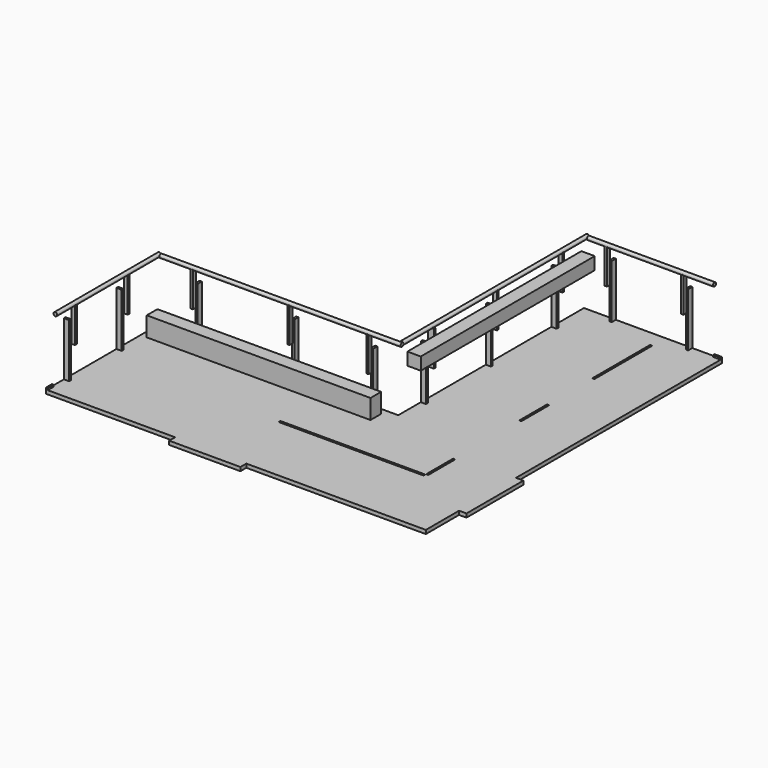
from build123d import *

# Parameters (mm, degrees)
F1_DEPTH  = 25.4
F2_W      = 30
F2_H      = 70
F2_W_2    = 70
F2_H_2    = 30
F3_DEPTH  = 750
F5_W      = 50
F5_H      = 30
F6_DEPTH  = 470
F5_W_2    = 30
F5_H_2    = 50
F7_R      = 25
F8_DEPTH  = 1700
F9_R      = 25
F10_DEPTH = 3130
F11_R     = 25
F12_DEPTH = 3250
F13_R     = 25
F14_DEPTH = 1750
F16_W     = 25
F16_H     = 970
F17_DEPTH = 3
F16_H_2   = 465
F16_W_2   = 1950
F16_H_3   = 25
F16_H_4   = 450
F18_DEPTH = 25
F19_W     = 100
F19_H     = 22
F19_W_2   = 22
F19_H_2   = 100
F20_DEPTH = 25
F21_DEPTH = 25
F22_W     = 2931.857542173
F22_H     = 168.5780864702
F23_DEPTH = 180
F24_W     = 3016.7315006256
F24_H     = 261.820666492
F25_DEPTH = 180


with BuildPart() as f1:
    # F0 (on Top) → F1 (new body)
    with BuildSketch(Plane.XY):
        Polygon((-2420, 0), (0, 0), (0, 560), (100, 560), (100, 1520), (0, 1520), (0, 4990), (-1860, 4990), (-1860, 1860), (-5120, 1860), (-5120, 0), (-3380, 0), (-3380, -100), (-2420, -100), align=None)
    extrude(amount=F1_DEPTH)

    # F2 (on face) → F3 (join)
    with BuildSketch(Plane.XY.offset(25.4)):
        with Locations((-415, 4955)):
            Rectangle(F2_W, F2_H)
        with Locations((-1825, 4455)):
            Rectangle(F2_W_2, F2_H_2)
        with Locations((-1825, 2255)):
            Rectangle(F2_W_2, F2_H_2)
        with Locations((-2156.2518024445, 1825)):
            Rectangle(F2_W, F2_H)
        with Locations((-3220.6851100922, 1825)):
            Rectangle(F2_W, F2_H)
        with Locations((-4523.8569831848, 1825)):
            Rectangle(F2_W, F2_H)
        with Locations((-1445, 4955)):
            Rectangle(F2_W, F2_H)
        with Locations((-5085, 315)):
            Rectangle(F2_W_2, F2_H_2)
        with Locations((-1825, 3350)):
            Rectangle(F2_W_2, F2_H_2)
        with Locations((-5085, 1201.3461732864)):
            Rectangle(F2_W_2, F2_H_2)
    extrude(amount=F3_DEPTH)

    # F2 (on face) → F18 (join)
    with BuildSketch(Plane.XY.offset(25.4)):
        Polygon((-430, 4920), (-430, 4990), (-1430, 4990), (-1430, 4920), (-1460, 4920), (-1460, 4990), (-1860, 4990), (-1860, 4470), (-1790, 4470), (-1790, 4440), (-1860, 4440), (-1860, 3365), (-1790, 3365), (-1790, 3335), (-1860, 3335), (-1860, 2270), (-1790, 2270), (-1790, 2240), (-1860, 2240), (-1860, 1860), (-2141.2518024445, 1860), (-2141.2518024445, 1790), (-2171.2518024445, 1790), (-2171.2518024445, 1860), (-3205.6851100922, 1860), (-3205.6851100922, 1790), (-3235.6851100922, 1790), (-3235.6851100922, 1860), (-4508.8569831848, 1860), (-4508.8569831848, 1790), (-4538.8569831848, 1790), (-4538.8569831848, 1860), (-5120, 1860), (-5120, 1216.3461732864), (-5050, 1216.3461732864), (-5050, 1186.3461732864), (-5120, 1186.3461732864), (-5120, 330), (-5050, 330), (-5050, 300), (-5120, 300), (-5120, 0), (-3380, 0), (-3380, -100), (-2420, -100), (-2420, 0), (0, 0), (0, 560), (100, 560), (100, 1520), (0, 1520), (0, 4990), (-400, 4990), (-400, 4920), align=None)
    extrude(amount=F18_DEPTH)

    # F19 (on face) → F20 (join)
    with BuildSketch(Plane.XY.offset(50.4)):
        with Locations((-50, 4979)):
            Rectangle(F19_W, F19_H)
        with Locations((-5109, 50)):
            Rectangle(F19_W_2, F19_H_2)
    extrude(amount=F20_DEPTH)


with BuildPart() as f6:
    # F5 (on offset) → F6 (new body)
    with BuildSketch(Plane.XY.offset(505.4)):
        with Locations((-1735, 4455)):
            Rectangle(F5_W, F5_H)
    extrude(amount=F6_DEPTH)



with BuildPart() as f6b:
    # F5 (on offset) → F6, piece 2 (new body)
    with BuildSketch(Plane.XY.offset(505.4)):
        with Locations((-1445, 4865)):
            Rectangle(F5_W_2, F5_H_2)
    extrude(amount=F6_DEPTH)



with BuildPart() as f6c:
    # F5 (on offset) → F6, piece 3 (new body)
    with BuildSketch(Plane.XY.offset(505.4)):
        with Locations((-415, 4865)):
            Rectangle(F5_W_2, F5_H_2)
    extrude(amount=F6_DEPTH)


with BuildPart() as f6d:
    # F5 (on offset) → F6, piece 4 (new body)
    with BuildSketch(Plane.XY.offset(505.4)):
        with Locations((-1735, 2255)):
            Rectangle(F5_W, F5_H)
    extrude(amount=F6_DEPTH)


with BuildPart() as f6e:
    # F5 (on offset) → F6, piece 5 (new body)
    with BuildSketch(Plane.XY.offset(505.4)):
        with Locations((-2156.2518024445, 1735)):
            Rectangle(F5_W_2, F5_H_2)
    extrude(amount=F6_DEPTH)



with BuildPart() as f6f:
    # F5 (on offset) → F6, piece 6 (new body)
    with BuildSketch(Plane.XY.offset(505.4)):
        with Locations((-3220.6851100922, 1735)):
            Rectangle(F5_W_2, F5_H_2)
    extrude(amount=F6_DEPTH)


with BuildPart() as f6g:
    # F5 (on offset) → F6, piece 7 (new body)
    with BuildSketch(Plane.XY.offset(505.4)):
        with Locations((-4523.8569831848, 1735)):
            Rectangle(F5_W_2, F5_H_2)
    extrude(amount=F6_DEPTH)


with BuildPart() as f6h:
    # F5 (on offset) → F6, piece 8 (new body)
    with BuildSketch(Plane.XY.offset(505.4)):
        with Locations((-4995, 315)):
            Rectangle(F5_W, F5_H)
    extrude(amount=F6_DEPTH)



with BuildPart() as f6i:
    # F5 (on offset) → F6, piece 9 (new body)
    with BuildSketch(Plane.XY.offset(505.4)):
        with Locations((-4995, 1201.3461732864)):
            Rectangle(F5_W, F5_H)
    extrude(amount=F6_DEPTH)


with BuildPart() as f6j:
    # F5 (on offset) → F6, piece 10 (new body)
    with BuildSketch(Plane.XY.offset(505.4)):
        with Locations((-1735, 3350)):
            Rectangle(F5_W, F5_H)
    extrude(amount=F6_DEPTH)


with BuildPart() as f6b_1:
    add(f6b.part)

    add(f6c.part)  # F8 merges F6c
    # F7 (on face) → F8 (join)
    with BuildSketch(Plane.YZ):
        with Locations((4865, 985.4)):
            Circle(F7_R)
    extrude(amount=-F8_DEPTH)


with BuildPart() as f6_1:
    add(f6.part)

    add(f6d.part)  # F10 merges F6d

    add(f6j.part)  # F10 merges F6j
    # F9 (on face) → F10 (join)
    with BuildSketch(Plane(origin=(0, 4890, 0), x_dir=(-1, 0, 0), z_dir=(0, 1, 0))):
        with Locations((1735, 985.4)):
            Circle(F9_R)
    extrude(amount=-F10_DEPTH)

    # F21 (add): a face of the model
    f21_faces = [f6_1.faces().sort_by_distance(p)[0] for p in [
        (-1710, 2255, 740.4),
    ]]
    extrude(f21_faces, amount=F21_DEPTH)

    # F22 (on face) → F23 (join)
    with BuildSketch(Plane.YZ.offset(-1685)):
        with Locations((3261.6109848022, 804.6890432351)):
            Rectangle(F22_W, F22_H)
    extrude(amount=F23_DEPTH)


with BuildPart() as f6e_1:
    add(f6e.part)

    add(f6f.part)  # F12 merges F6f

    add(f6g.part)  # F12 merges F6g
    # F11 (on face) → F12 (join)
    with BuildSketch(Plane.YZ.offset(-1710)):
        with Locations((1735, 985.4)):
            Circle(F11_R)
    extrude(amount=-F12_DEPTH)


with BuildPart() as f6h_1:
    add(f6h.part)

    add(f6i.part)  # F14 merges F6i
    # F13 (on face) → F14 (join)
    with BuildSketch(Plane.XZ):
        with Locations((-4995, 985.4)):
            Circle(F13_R)
    extrude(amount=-F14_DEPTH)


with BuildPart() as f17:
    # F16 (on offset) → F17 (new body)
    with BuildSketch(Plane.XY.offset(685.4)):
        with Locations((-12.5, 3325)):
            Rectangle(F16_W, F16_H)
    extrude(amount=F17_DEPTH)


with BuildPart() as f17b:
    # F16 (on offset) → F17, piece 2 (new body)
    with BuildSketch(Plane.XY.offset(685.4)):
        with Locations((-12.5, 1842.5)):
            Rectangle(F16_W, F16_H_2)
    extrude(amount=F17_DEPTH)


with BuildPart() as f17c:
    # F16 (on offset) → F17, piece 3 (new body)
    with BuildSketch(Plane.XY.offset(685.4)):
        with Locations((-1005, 12.5)):
            Rectangle(F16_W_2, F16_H_3)
    extrude(amount=F17_DEPTH)


with BuildPart() as f17d:
    # F16 (on offset) → F17, piece 4 (new body)
    with BuildSketch(Plane.XY.offset(685.4)):
        with Locations((-12.5, 265)):
            Rectangle(F16_W, F16_H_4)
    extrude(amount=F17_DEPTH)


with BuildPart() as f25:
    # F24 (on face) → F25 (new body)
    with BuildSketch(Plane.XZ.offset(-1710)):
        with Locations((-3478.4697294235, 222.4028147757)):
            Rectangle(F24_W, F24_H)
    extrude(amount=F25_DEPTH)


solid = Compound([f1.part, f6b_1.part, f6_1.part, f6e_1.part, f6h_1.part, f17.part, f17b.part, f17c.part, f17d.part, f25.part])
